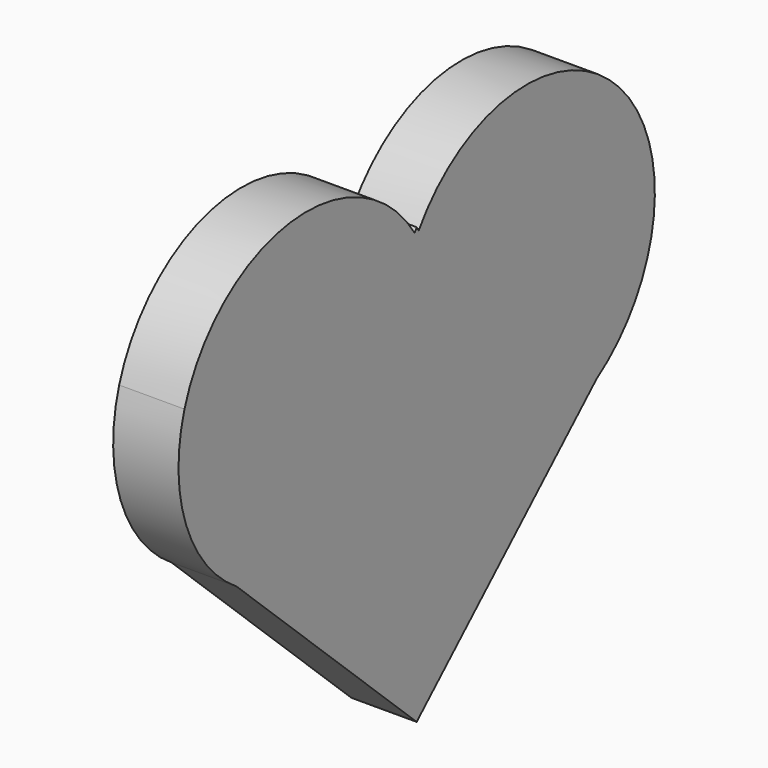
from build123d import *

# Parameters (mm, degrees)
F1_DEPTH = 4.7


# Not quite as in the source:
# - ends of sketch curves that miss each other by under 0.0002 mm in the source are joined


with BuildPart() as f1:
    # F0 (on Right) → F1 (new body)
    with BuildSketch(Plane.YZ):
        with BuildLine():
            ThreePointArc((-1.2861936627, 9.5404589046), (-1.3764412196, 9.3943245755), (-1.4645028348, 9.2468626631))
            ThreePointArc((-1.4645028348, 9.2468626631), (-12.6873926867, 14.4502544968), (-22.1664207404, 6.501885459))
            ThreePointArc((-22.1664207404, 6.501885459), (-22.0324514747, -0.8678048449), (-17.463284327, -6.6516612154))
            add(Edge.make_bspline(
                [(-17.463284327, -6.6516612154), (-12.0709199928, -11.7001523748), (-6.6785564381, -16.7486430269), (-1.2861928833, -21.797133679)],
                knots=[0, 0, 0, 0, 22.160405753, 22.160405753, 22.160405753, 22.160405753], degree=3))
            add(Edge.make_bspline(
                [(14.8908962222, -6.6516617227), (9.4985326674, -11.7001523748), (4.1061691126, -16.7486430269), (-1.2861928833, -21.797133679)],
                knots=[0, 0, 0, 0, 22.160405753, 22.160405753, 22.160405753, 22.160405753], degree=3))
            ThreePointArc((14.8908962222, -6.6516617227), (19.4600641493, -0.8678048449), (19.594033415, 6.501885459))
            ThreePointArc((19.594033415, 6.501885459), (10.1150053613, 14.4502544968), (-1.1078844907, 9.2468626631))
            ThreePointArc((-1.1078844907, 9.2468626631), (-1.1959461058, 9.3943245755), (-1.2861936627, 9.5404589046))
        make_face()
    extrude(amount=F1_DEPTH)


solid = f1.part
